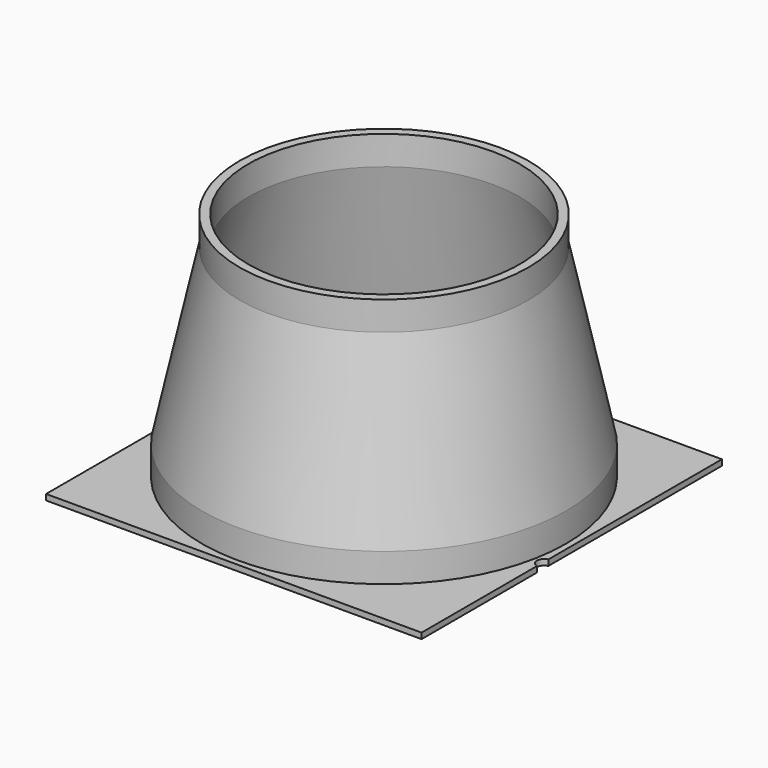
from build123d import *

# Parameters (mm, degrees)
F0_R     = 63
F0_R_2   = 60
F1_DEPTH = 2
F2_DEPTH = 12
F5_DEPTH = 10


with BuildPart() as f1:
    # F0 (on Top) → F1 (new body)
    with BuildSketch(Plane.XY):
        with BuildLine():
            Line((65, 65), (-65, 65))
            Line((-65, 65), (-65, -65))
            Line((-65, -65), (65, -65))
            Line((65, -65), (65, -15.0111682118))
            ThreePointArc((65, -15.0111682118), (63.0170909154, -12.5652293358), (65, -10.1192904598))
            Line((65, -10.1192904598), (65, 65))
        make_face()
        Circle(F0_R, mode=Mode.SUBTRACT)
        Circle(F0_R)
        Circle(F0_R_2, mode=Mode.SUBTRACT)
    extrude(amount=F1_DEPTH)

    # F0 (on Top) → F2 (join)
    with BuildSketch(Plane.XY):
        Circle(F0_R)
        Circle(F0_R_2, mode=Mode.SUBTRACT)
    extrude(amount=F2_DEPTH)

    # F3 (on Right) → F4 (revolve)
    with BuildSketch(Plane.YZ):
        Polygon((47, 72), (60, 12), (63, 12), (50, 72), align=None)
    revolve(axis=Axis((0, 0, 42), (0, 0, 1)))

    # F5 (add): a face of the model
    f5_faces = [f1.faces().sort_by_distance(p)[0] for p in [
        (0, -48.5857864376, 72),
    ]]
    extrude(f5_faces, amount=F5_DEPTH)


solid = f1.part
